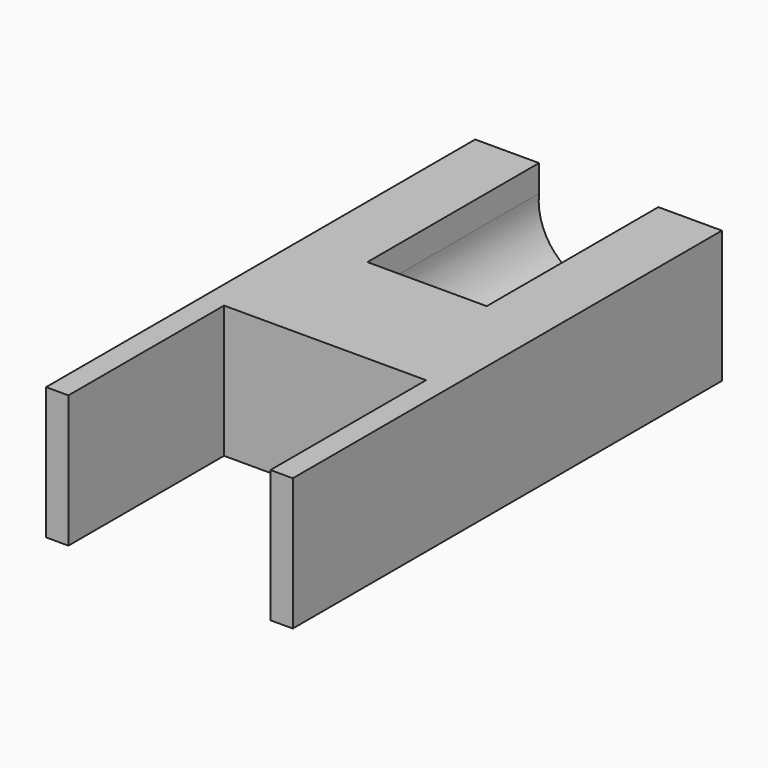
from build123d import *

# Parameters (mm, degrees)
F1_DEPTH = 9.398
F3_DEPTH = 15.24


with BuildPart() as f1:
    # F0 (on Top) → F1 (new body)
    with BuildSketch(Plane.XY):
        Polygon((0, 38.1), (0, 0), (1.5875, 0), (1.5875, 13.8176), (15.9385, 13.8176), (15.9385, 0), (17.526, 0), (17.526, 38.1), align=None)
    extrude(amount=F1_DEPTH)

    # F2 (on face) → F3 (cut)
    with BuildSketch(Plane(origin=(0, 38.1, 0), x_dir=(-1, 0, 0), z_dir=(0, 1, 0))):
        with BuildLine():
            Line((-13.0094570703, 9.398), (-13.0094570703, 7.2687586724))
            ThreePointArc((-13.0094570703, 7.2687586724), (-8.647429717, 2.7979053307), (-4.5347851701, 7.4991782504))
            Line((-4.5347851701, 7.4991782504), (-4.5347851701, 9.398))
            Line((-4.5347851701, 9.398), (-13.0094570703, 9.398))
        make_face()
    extrude(amount=-F3_DEPTH, mode=Mode.SUBTRACT)


solid = f1.part
